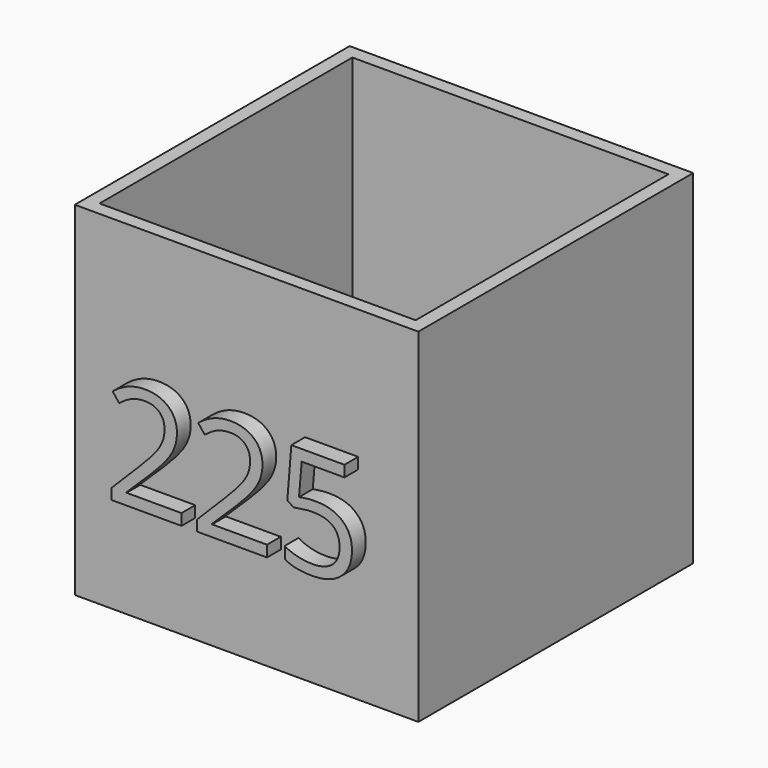
from build123d import *

# Parameters (mm, degrees)
F0_W         = 20
F0_H         = 20
F1_DEPTH     = 20
F2_T         = -0.8
F3_TEXT_SIZE = 8.7082728592
F4_DEPTH     = 1


# Not quite as in the source:
# - Text() gives the source's letters only with a copy of the font that has no kerning and outlines rounded to 1/6400 em; it was checked with that copy


with BuildPart() as f1:
    # F0 (on Top) → F1 (new body)
    with BuildSketch(Plane.XY):
        Rectangle(F0_W, F0_H)
    extrude(amount=F1_DEPTH)

    # F2
    f2_openings = [f1.faces().sort_by_distance(p)[0] for p in [
        (0, 0, 20),
    ]]
    offset(amount=F2_T, openings=f2_openings)

    # F3 (on face) → F4 (join)
    with BuildSketch(Plane.XZ.offset(10)):
        with Locations((-7.5, 6.2300435414)):
            Text('225', F3_TEXT_SIZE, font='Open Sans', text_align=(TextAlign.LEFT, TextAlign.BOTTOM))
    extrude(amount=F4_DEPTH)


solid = f1.part
